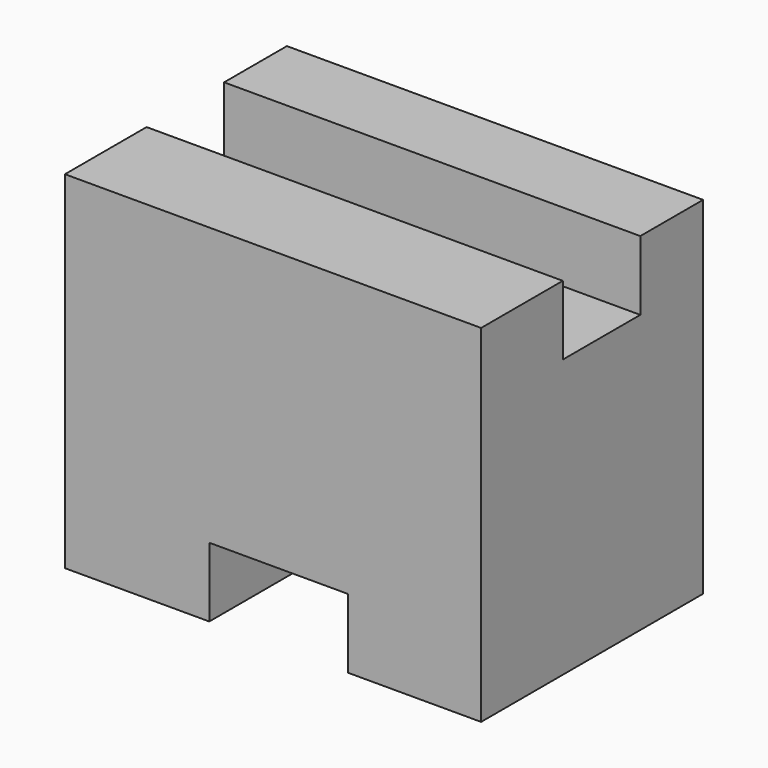
from build123d import *

# Parameters (mm, degrees)
F0_W     = 38.1
F0_H     = 31.75
F1_DEPTH = 25.4
F2_W     = 12.7
F2_H     = 6.35
F3_DEPTH = 25.401
F4_W     = 38.1
F4_H     = 8.8702891953
F5_DEPTH = 6.35


# Not quite as in the source:
# - a length typed as a fraction of an inch, garbled in the dataset ("3 / 203.2 mm" for 3/8 in), is restored


with BuildPart() as f1:
    # F0 (on Front) → F1 (new body)
    with BuildSketch(Plane.XZ):
        with Locations((19.05, 15.875)):
            Rectangle(F0_W, F0_H)
    extrude(amount=F1_DEPTH)

    # F2 (on face) → F3 (cut, through all)
    with BuildSketch(Plane.XZ.offset(25.4)):
        with Locations((19.5667292759, 3.175)):
            Rectangle(F2_W, F2_H)
    extrude(amount=-F3_DEPTH, mode=Mode.SUBTRACT)

    # F4 (on face) → F5 (cut)
    with BuildSketch(Plane.XY.offset(31.75)):
        with Locations((19.05, -11.620078003)):
            Rectangle(F4_W, F4_H)
    extrude(amount=-F5_DEPTH, mode=Mode.SUBTRACT)


solid = f1.part
